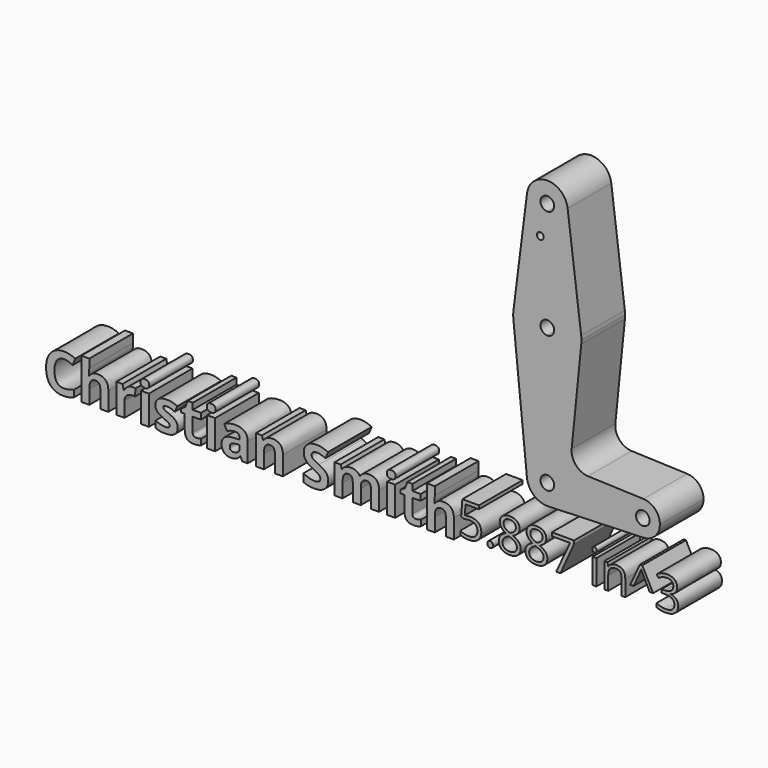
from build123d import *

# Parameters (mm, degrees)
F0_R           = 1.5875
F0_TEXT_SIZE   = 21.7160856765
F0_TEXT_SIZE_2 = 24.9441273303
F1_DEPTH       = 25.4


# Not quite as in the source:
# - Text() gives the source's letters only with a copy of the font that has no kerning and outlines rounded to 1/6400 em; it was checked with that copy


with BuildPart() as f1:
    # F0 (on Front) → F1 (new body)
    with BuildSketch(Plane.XZ):
        with BuildLine():
            ThreePointArc((-96.3130220771, 56.9771687746), (-89.5778299863, 59.7669766838), (-86.7880220771, 66.5021687746))
            ThreePointArc((-86.7880220771, 66.5021687746), (-86.8067171829, 67.0986520166), (-86.8627291129, 67.6927937746))
            ThreePointArc((-86.8627291129, 67.6927937746), (-96.3130220771, 76.0271687746), (-105.7633150413, 67.6927937746))
            ThreePointArc((-105.7633150413, 67.6927937746), (-103.4567720771, 60.2019734651), (-96.3130220771, 56.9771687746))
        make_face()
        with BuildLine():
            ThreePointArc((-93.1380220771, 66.5021687746), (-94.0679580468, 64.2571047443), (-96.3130220771, 63.3271687746))
            ThreePointArc((-96.3130220771, 63.3271687746), (-98.5580861074, 68.7472328049), (-93.1380220771, 66.5021687746))
        make_face(mode=Mode.SUBTRACT)
        with BuildLine():
            ThreePointArc((-86.8627291129, 67.6927937746), (-86.8067171829, 67.0986520166), (-86.7880220771, 66.5021687746))
            ThreePointArc((-86.7880220771, 66.5021687746), (-89.5778299863, 59.7669766838), (-96.3130220771, 56.9771687746))
            Line((-96.3130220771, 56.9771687746), (-96.3130220771, 52.2273687746))
            Line((-96.3130220771, 52.2273687746), (-96.3130220771, 31.5771687746))
            ThreePointArc((-96.3130220771, 31.5771687746), (-85.8126965613, 27.6084187746), (-80.5625338034, 17.6865437746))
            Line((-80.5625338034, 17.6865437746), (-86.8627291129, 67.6927937746))
        make_face()
        with BuildLine():
            Line((-96.3130220771, 52.2273687746), (-96.3130220771, 56.9771687746))
            ThreePointArc((-96.3130220771, 56.9771687746), (-103.4567720771, 60.2019734651), (-105.7633150413, 67.6927937746))
            Line((-105.7633150413, 67.6927937746), (-112.0635103508, 17.6865437746))
            ThreePointArc((-112.0635103508, 17.6865437746), (-106.8133475929, 27.6084187746), (-96.3130220771, 31.5771687746))
            Line((-96.3130220771, 31.5771687746), (-96.3130220771, 52.2273687746))
        make_face()
        with Locations((-99.575035274, 52.2273687746)):
            Circle(F0_R, mode=Mode.SUBTRACT)
        with BuildLine():
            ThreePointArc((-80.4380220771, 15.7021687746), (-80.4691805867, 16.6963075112), (-80.5625338034, 17.6865437746))
            ThreePointArc((-80.5625338034, 17.6865437746), (-85.8126965613, 27.6084187746), (-96.3130220771, 31.5771687746))
            Line((-96.3130220771, 31.5771687746), (-96.3130220771, 18.8771687746))
            ThreePointArc((-96.3130220771, 18.8771687746), (-94.0679580468, 17.9472328049), (-93.1380220771, 15.7021687746))
            ThreePointArc((-93.1380220771, 15.7021687746), (-94.0679580468, 13.4571047443), (-96.3130220771, 12.5271687746))
            Line((-96.3130220771, 12.5271687746), (-96.3130220771, -0.1728312254))
            ThreePointArc((-96.3130220771, -0.1728312254), (-85.6637483342, 3.9289536763), (-80.517596513, 14.1146687746))
            ThreePointArc((-80.517596513, 14.1146687746), (-80.4579281665, 14.9074222205), (-80.4380220771, 15.7021687746))
        make_face()
        with BuildLine():
            ThreePointArc((-96.3130220771, 31.5771687746), (-106.8133475929, 27.6084187746), (-112.0635103508, 17.6865437746))
            ThreePointArc((-112.0635103508, 17.6865437746), (-112.1867658925, 15.9018742613), (-112.1084476412, 14.1146687746))
            ThreePointArc((-112.1084476412, 14.1146687746), (-106.9622958199, 3.9289536763), (-96.3130220771, -0.1728312254))
            Line((-96.3130220771, -0.1728312254), (-96.3130220771, 12.5271687746))
            ThreePointArc((-96.3130220771, 12.5271687746), (-99.4880220771, 15.7021687746), (-96.3130220771, 18.8771687746))
            Line((-96.3130220771, 18.8771687746), (-96.3130220771, 31.5771687746))
        make_face()
        with BuildLine():
            ThreePointArc((-96.3130220771, -0.1728312254), (-106.9622958199, 3.9289536763), (-112.1084476412, 14.1146687746))
            Line((-112.1084476412, 14.1146687746), (-105.7902774155, -48.7503312254))
            ThreePointArc((-105.7902774155, -48.7503312254), (-103.376951136, -41.4082669797), (-96.3130220771, -38.2728312254))
            Line((-96.3130220771, -38.2728312254), (-96.3130220771, -0.1728312254))
        make_face()
        with BuildLine():
            Line((-84.9718354848, -30.204449413), (-80.517596513, 14.1146687746))
            ThreePointArc((-80.517596513, 14.1146687746), (-85.6637483342, 3.9289536763), (-96.3130220771, -0.1728312254))
            Line((-96.3130220771, -0.1728312254), (-96.3130220771, -38.2728312254))
            ThreePointArc((-96.3130220771, -38.2728312254), (-89.5778299863, -41.0626391346), (-86.7880220771, -47.7978312254))
            Line((-86.7880220771, -47.7978312254), (-59.8005220771, -47.7978312254))
            ThreePointArc((-59.8005220771, -47.7978312254), (-57.3745448585, -42.0858243207), (-51.5795399342, -39.8653950218))
            Line((-51.5795399342, -39.8653950218), (-77.3454220766, -38.9445975146))
            ThreePointArc((-77.3454220766, -38.9445975146), (-83.0518221797, -36.2264720755), (-84.9718354848, -30.204449413))
        make_face()
        with BuildLine():
            ThreePointArc((-96.3130220771, -38.2728312254), (-103.376951136, -41.4082669797), (-105.7902774155, -48.7503312254))
            ThreePointArc((-105.7902774155, -48.7503312254), (-102.5754054587, -54.9747511345), (-95.9728435057, -57.3167546698))
            ThreePointArc((-95.9728435057, -57.3167546698), (-89.4586137914, -54.4116585631), (-86.7880220771, -47.7978312254))
            Line((-86.7880220771, -47.7978312254), (-93.1380220771, -47.7978312254))
            ThreePointArc((-93.1380220771, -47.7978312254), (-98.5580861074, -50.0428952557), (-96.3130220771, -44.6228312254))
            Line((-96.3130220771, -44.6228312254), (-96.3130220771, -38.2728312254))
        make_face()
        with BuildLine():
            ThreePointArc((-86.7880220771, -47.7978312254), (-89.4586137914, -54.4116585631), (-95.9728435057, -57.3167546698))
            Line((-95.9728435057, -57.3167546698), (-51.5795399342, -55.730267429))
            ThreePointArc((-51.5795399342, -55.730267429), (-57.3745448585, -53.5098381301), (-59.8005220771, -47.7978312254))
            Line((-59.8005220771, -47.7978312254), (-86.7880220771, -47.7978312254))
        make_face()
        with BuildLine():
            ThreePointArc((-59.8005220771, -47.7978312254), (-57.3745448585, -53.5098381301), (-51.5795399342, -55.730267429))
            ThreePointArc((-51.5795399342, -55.730267429), (-46.1510151724, -53.3093540069), (-43.9255220771, -47.7978312254))
            ThreePointArc((-43.9255220771, -47.7978312254), (-46.1510151724, -42.2863084439), (-51.5795399342, -39.8653950218))
            ThreePointArc((-51.5795399342, -39.8653950218), (-57.3745448585, -42.0858243207), (-59.8005220771, -47.7978312254))
        make_face()
        with BuildLine():
            ThreePointArc((-48.6880220771, -47.7978312254), (-51.8630220771, -50.9728312254), (-55.0380220771, -47.7978312254))
            ThreePointArc((-55.0380220771, -47.7978312254), (-51.8630220771, -44.6228312254), (-48.6880220771, -47.7978312254))
        make_face(mode=Mode.SUBTRACT)
        with Locations((-138.1975290254, -82.8736014664)):
            Text('5.887 in^3', F0_TEXT_SIZE, font='Open Sans', text_align=(TextAlign.LEFT, TextAlign.BOTTOM))
        with Locations((-331.0078382492, -85.1977914572)):
            Text('Christian Smith', F0_TEXT_SIZE_2, font='Open Sans', font_style=FontStyle.BOLD, text_align=(TextAlign.LEFT, TextAlign.BOTTOM))
        with BuildLine():
            ThreePointArc((-86.7880220771, -47.7978312254), (-89.5778299863, -41.0626391346), (-96.3130220771, -38.2728312254))
            Line((-96.3130220771, -38.2728312254), (-96.3130220771, -44.6228312254))
            ThreePointArc((-96.3130220771, -44.6228312254), (-94.0679580468, -45.5527671951), (-93.1380220771, -47.7978312254))
            Line((-93.1380220771, -47.7978312254), (-86.7880220771, -47.7978312254))
        make_face()
    extrude(amount=F1_DEPTH)


solid = f1.part
